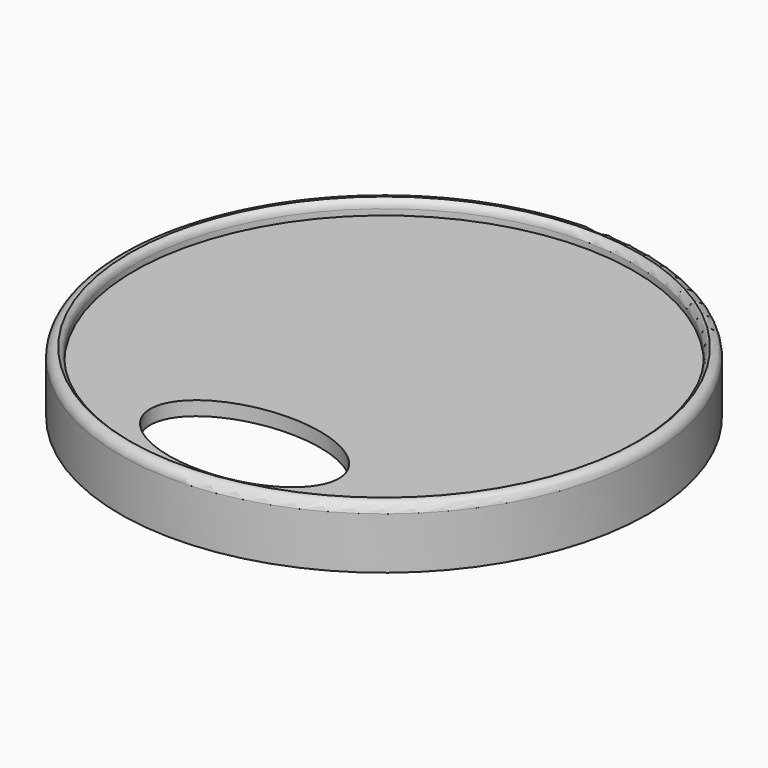
from build123d import *

# Parameters (mm, degrees)
F0_R     = 28
F1_DEPTH = 5
F2_R     = 26
F3_DEPTH = 3.5
F4_R     = 26.5
F5_DEPTH = 2
F7_DEPTH = 6
F8_R     = 28
F8_R_2   = 26.5
F9_DEPTH = 1.5
F10_R    = 1


# Not quite as in the source:
# - a fillet or chamfer that OpenCascade refuses, or shapes differently, is made with other operations: its cross-section is extruded or revolved along the edge and cut away or added


with BuildPart() as f1:
    # F0 (on Top) → F1 (new body)
    with BuildSketch(Plane.XY):
        Circle(F0_R)
    extrude(amount=F1_DEPTH)

    # F2 (on face) → F3 (cut)
    with BuildSketch(Plane(origin=(0, 0, 0), x_dir=(1, 0, 0), z_dir=(0, 0, -1))):
        Circle(F2_R)
    extrude(amount=-F3_DEPTH, mode=Mode.SUBTRACT)

    # F4 (on face) → F5 (cut)
    with BuildSketch(Plane(origin=(0, 0, 3.5), x_dir=(1, 0, 0), z_dir=(0, 0, -1))):
        Circle(F4_R)
    extrude(amount=F5_DEPTH, mode=Mode.SUBTRACT)

    # F6 (on face) → F7 (cut)
    with BuildSketch(Plane.XY.offset(5)):
        with BuildLine():
            add(Edge.make_bspline(
                [(-10, -18.4983219951), (-10, -28.8906268406), (5, -23.6944744178), (20, -18.4983219951), (5, -13.3021695724), (-10, -8.1060171497), (-10, -18.4983219951)],
                knots=[0, 0, 0, 2.0943951024, 2.0943951024, 4.1887902048, 4.1887902048, 6.2831853072, 6.2831853072, 6.2831853072], degree=2, weights=[1, 0.5, 1, 0.5, 1, 0.5, 1]))
        make_face()
    extrude(amount=-F7_DEPTH, mode=Mode.SUBTRACT)

    # F8 (on face) → F9 (join)
    with BuildSketch(Plane.XY.offset(5)):
        Circle(F8_R)
        Circle(F8_R_2, mode=Mode.SUBTRACT)
    extrude(amount=F9_DEPTH)

    # F10
    f10_edges = [f1.edges().sort_by_distance(p)[0] for p in [
        (-28, 0, 6.5),
    ]]
    fillet(f10_edges, radius=F10_R)

    # F11: fillet of radius 1 on 1 edges, made by hand

    # F11_s1 → F11_t2 (revolve, cut)
    with BuildSketch(Plane.XZ):
        with BuildLine():
            ThreePointArc((27, 6.5), (26.6339745962, 6.1339745962), (26.5, 5.6339745962))
            Line((26.5, 5.6339745962), (26.48, 5.6339745962))
            Line((26.48, 5.6339745962), (26.48, 6.5))
            Line((26.48, 6.5), (26.5, 6.52))
            ThreePointArc((26.5, 6.52), (26.75, 6.52), (26.99, 6.5173205081))
            Line((26.99, 6.5173205081), (27, 6.5))
        make_face()
    revolve(axis=Axis((0, 0, 6.5), (0, 0, 1)), mode=Mode.SUBTRACT)


solid = f1.part
